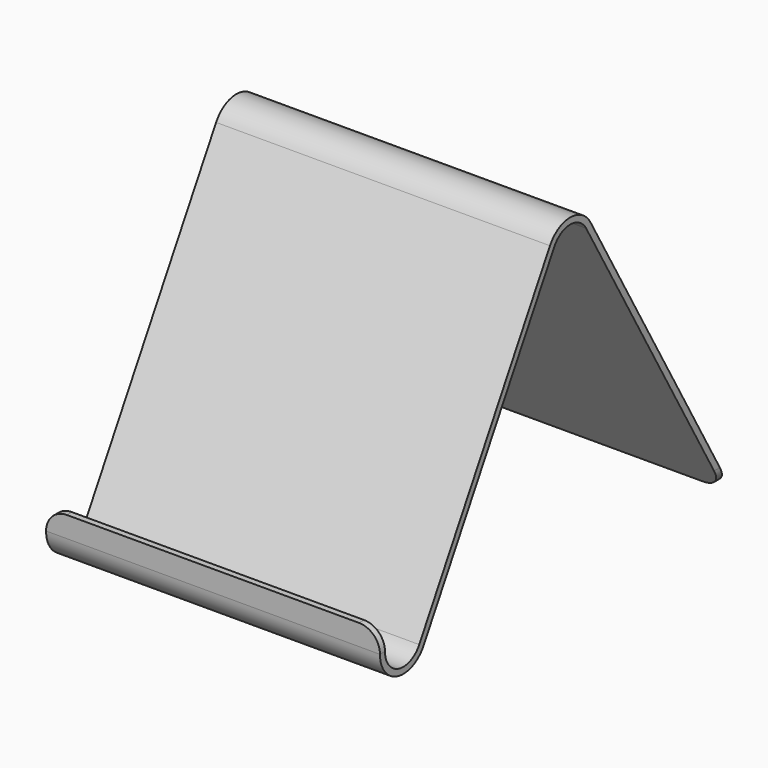
from build123d import *

# Parameters (mm, degrees)
F1_DEPTH    = 40
F2_T1_DEPTH = 14
F2_T3_DEPTH = 26.7295341336


# Not quite as in the source:
# - a fillet or chamfer that OpenCascade refuses, or shapes differently, is made with other operations: its cross-section is extruded or revolved along the edge and cut away or added


with BuildPart() as f1:
    # F0 (on Right) → F1 (new body, symmetric)
    with BuildSketch(Plane.YZ):
        with BuildLine():
            Line((-7, 5), (-7, 0))
            ThreePointArc((-7, 0), (-1.8031925829, -6.7637634871), (6.0709990026, -3.484676615))
            Line((6.0709990026, -3.484676615), (45.2299293551, 64.7379601975))
            ThreePointArc((45.2299293551, 64.7379601975), (50, 67.5), (54.7700706449, 64.7379601975))
            Line((54.7700706449, 64.7379601975), (95.9467521433, -7))
            Line((95.9467521433, -7), (97.6762862769, -7))
            Line((97.6762862769, -7), (56.0709990026, 65.484676615))
            ThreePointArc((56.0709990026, 65.484676615), (50, 69), (43.9290009974, 65.484676615))
            Line((43.9290009974, 65.484676615), (4.7700706449, -2.7379601975))
            ThreePointArc((4.7700706449, -2.7379601975), (-1.4167941723, -5.314385597), (-5.5, 0))
            Line((-5.5, 0), (-5.5, 5))
            Line((-5.5, 5), (-7, 5))
        make_face()
    extrude(amount=F1_DEPTH, both=True)

    # F2: fillet of radius 5 on 4 edges, made by hand

    # F2_s2 → F2_t1 (cut)
    with BuildSketch(Plane.XZ.offset(5.5)):
        with BuildLine():
            ThreePointArc((35, 5), (38.5355339059, 3.5355339059), (40, 0))
            Line((40, 0), (40, 5))
            Line((40, 5), (35, 5))
        make_face()
        with BuildLine():
            ThreePointArc((-35, 5), (-38.5355339059, 3.5355339059), (-40, 0))
            Line((-40, 0), (-40, 5))
            Line((-40, 5), (-35, 5))
        make_face()
    extrude(amount=F2_T1_DEPTH, mode=Mode.SUBTRACT)

    # F2_s4 → F2_t3 (cut)
    with BuildSketch(Plane.XZ.offset(-110.1762862769)):
        with BuildLine():
            ThreePointArc((35, -7), (38.5355339059, -5.5355339059), (40, -2))
            Line((40, -2), (40, -7))
            Line((40, -7), (35, -7))
        make_face()
        with BuildLine():
            ThreePointArc((-35, -7), (-38.5355339059, -5.5355339059), (-40, -2))
            Line((-40, -2), (-40, -7))
            Line((-40, -7), (-35, -7))
        make_face()
    extrude(amount=F2_T3_DEPTH, mode=Mode.SUBTRACT)


solid = f1.part
